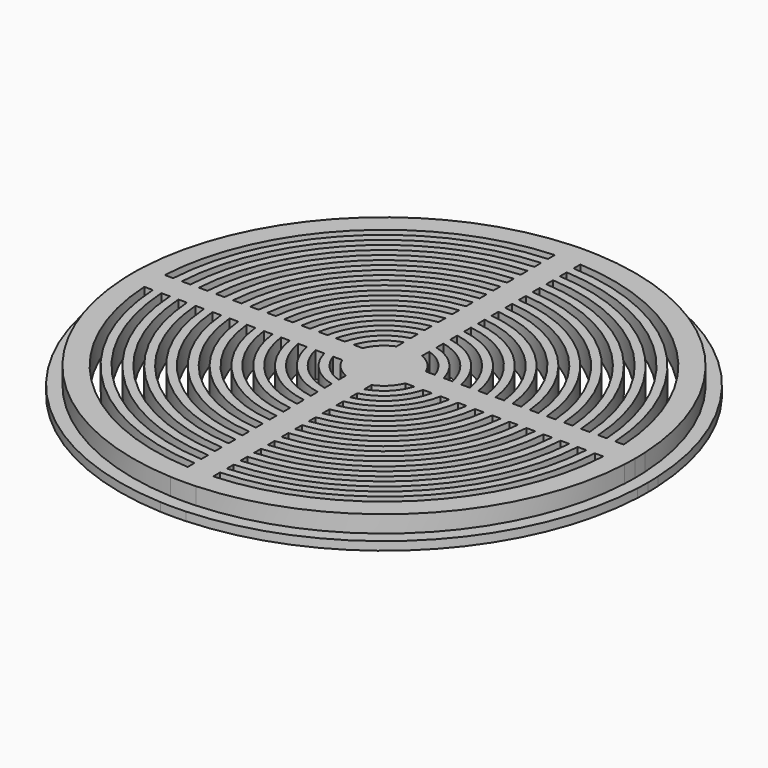
from build123d import *

# Parameters (mm, degrees)
F0_R     = 1
F1_DEPTH = 3
F2_DEPTH = 1


with BuildPart() as f1:
    # F0 (on Top) → F1 (new body)
    with BuildSketch(Plane.XY):
        with BuildLine():
            Line((-17.9373911147, 1.5), (-18.9406969249, 1.5))
            ThreePointArc((-18.9406969249, 1.5), (-19, 0), (-18.9406969249, -1.5))
            Line((-18.9406969249, -1.5), (-17.9373911147, -1.5))
            ThreePointArc((-17.9373911147, -1.5), (-18, 0), (-17.9373911147, 1.5))
        make_face()
        with BuildLine():
            Line((-11.9058808998, 1.5), (-12.9131715701, 1.5))
            ThreePointArc((-12.9131715701, 1.5), (-13, 0), (-12.9131715701, -1.5))
            Line((-12.9131715701, -1.5), (-11.9058808998, -1.5))
            ThreePointArc((-11.9058808998, -1.5), (-12, 0), (-11.9058808998, 1.5))
        make_face()
        with BuildLine():
            ThreePointArc((29.4618397253, -1.5), (29.4904583882, -0.7502426618), (29.5, 0))
            ThreePointArc((29.5, 0), (29.4904583882, 0.7502426618), (29.4618397253, 1.5))
            Line((29.4618397253, 1.5), (26.9583011334, 1.5))
            ThreePointArc((26.9583011334, 1.5), (26.9895732701, 0.7502897433), (27, 0))
            ThreePointArc((27, 0), (26.9895732701, -0.7502897433), (26.9583011334, -1.5))
            Line((26.9583011334, -1.5), (29.4618397253, -1.5))
        make_face()
        with BuildLine():
            ThreePointArc((26, 0), (25.9891714212, 0.750312493), (25.9566947048, 1.5))
            Line((25.9566947048, 1.5), (24.9549594269, 1.5))
            ThreePointArc((24.9549594269, 1.5), (24.9887373198, 0.7503380327), (25, 0))
            ThreePointArc((25, 0), (24.9887373198, -0.7503380327), (24.9549594269, -1.5))
            Line((24.9549594269, -1.5), (25.9566947048, -1.5))
            ThreePointArc((25.9566947048, -1.5), (25.9891714212, -0.750312493), (26, 0))
        make_face()
        with BuildLine():
            ThreePointArc((18, 0), (17.9843409674, 0.7506530278), (17.9373911147, 1.5))
            Line((17.9373911147, 1.5), (16.9336942219, 1.5))
            ThreePointArc((16.9336942219, 1.5), (16.9834154659, 0.7507323851), (17, 0))
            ThreePointArc((17, 0), (16.9834154659, -0.7507323851), (16.9336942219, -1.5))
            Line((16.9336942219, -1.5), (17.9373911147, -1.5))
            ThreePointArc((17.9373911147, -1.5), (17.9843409674, -0.7506530278), (18, 0))
        make_face()
        with BuildLine():
            Line((-19.9436706752, 1.5), (-20.9463600657, 1.5))
            ThreePointArc((-20.9463600657, 1.5), (-21, 0), (-20.9463600657, -1.5))
            Line((-20.9463600657, -1.5), (-19.9436706752, -1.5))
            ThreePointArc((-19.9436706752, -1.5), (-20, 0), (-19.9436706752, 1.5))
        make_face()
        with BuildLine():
            Line((-25.9566947048, 1.5), (-26.9583011334, 1.5))
            ThreePointArc((-26.9583011334, 1.5), (-27, 0), (-26.9583011334, -1.5))
            Line((-26.9583011334, -1.5), (-25.9566947048, -1.5))
            ThreePointArc((-25.9566947048, -1.5), (-26, 0), (-25.9566947048, 1.5))
        make_face()
        with BuildLine():
            Line((-1.5, 1.5), (-2.5980762114, 1.5))
            ThreePointArc((-2.5980762114, 1.5), (-3, 0), (-2.5980762114, -1.5))
            Line((-2.5980762114, -1.5), (-1.5, -1.5))
            Line((-1.5, -1.5), (-1.5, -1.3228756555))
            ThreePointArc((-1.5, -1.3228756555), (-2, 0), (-1.5, 1.3228756555))
            Line((-1.5, 1.3228756555), (-1.5, 1.5))
        make_face()
        with BuildLine():
            Line((-23.953079134, 1.5), (-24.9549594269, 1.5))
            ThreePointArc((-24.9549594269, 1.5), (-25, 0), (-24.9549594269, -1.5))
            Line((-24.9549594269, -1.5), (-23.953079134, -1.5))
            ThreePointArc((-23.953079134, -1.5), (-24, 0), (-23.953079134, 1.5))
        make_face()
        with BuildLine():
            Line((-21.9488040676, 1.5), (-22.9510348351, 1.5))
            ThreePointArc((-22.9510348351, 1.5), (-23, 0), (-22.9510348351, -1.5))
            Line((-22.9510348351, -1.5), (-21.9488040676, -1.5))
            ThreePointArc((-21.9488040676, -1.5), (-22, 0), (-21.9488040676, 1.5))
        make_face()
        with BuildLine():
            ThreePointArc((5, 0), (4.9420886291, 0.7587884964), (4.7696960071, 1.5))
            Line((4.7696960071, 1.5), (3.7080992435, 1.5))
            ThreePointArc((3.7080992435, 1.5), (3.92634671, 0.7640690498), (4, 0))
            ThreePointArc((4, 0), (3.92634671, -0.7640690498), (3.7080992435, -1.5))
            Line((3.7080992435, -1.5), (4.7696960071, -1.5))
            ThreePointArc((4.7696960071, -1.5), (4.9420886291, -0.7587884964), (5, 0))
        make_face()
        with BuildLine():
            Line((-7.8581168228, 1.5), (-8.8741196746, 1.5))
            ThreePointArc((-8.8741196746, 1.5), (-9, 0), (-8.8741196746, -1.5))
            Line((-8.8741196746, -1.5), (-7.8581168228, -1.5))
            ThreePointArc((-7.8581168228, -1.5), (-8, 0), (-7.8581168228, 1.5))
        make_face()
        with BuildLine():
            Line((-13.9194109071, 1.5), (-14.9248115566, 1.5))
            ThreePointArc((-14.9248115566, 1.5), (-15, 0), (-14.9248115566, -1.5))
            Line((-14.9248115566, -1.5), (-13.9194109071, -1.5))
            ThreePointArc((-13.9194109071, -1.5), (-14, 0), (-13.9194109071, 1.5))
        make_face()
        with BuildLine():
            Line((-15.9295323221, 1.5), (-16.9336942219, 1.5))
            ThreePointArc((-16.9336942219, 1.5), (-17, 0), (-16.9336942219, -1.5))
            Line((-16.9336942219, -1.5), (-15.9295323221, -1.5))
            ThreePointArc((-15.9295323221, -1.5), (-16, 0), (-15.9295323221, 1.5))
        make_face()
        with BuildLine():
            Line((-5.8094750193, 1.5), (-6.8373971656, 1.5))
            ThreePointArc((-6.8373971656, 1.5), (-7, 0), (-6.8373971656, -1.5))
            Line((-6.8373971656, -1.5), (-5.8094750193, -1.5))
            ThreePointArc((-5.8094750193, -1.5), (-6, 0), (-5.8094750193, 1.5))
        make_face()
        with BuildLine():
            ThreePointArc((3, 0), (2.8977774789, 0.7764571353), (2.5980762114, 1.5))
            Line((2.5980762114, 1.5), (1.5, 1.5))
            Line((1.5, 1.5), (1.5, 1.3228756555))
            ThreePointArc((1.5, 1.3228756555), (1.8708286934, 0.7071067812), (2, 0))
            ThreePointArc((2, 0), (1.8708286934, -0.7071067812), (1.5, -1.3228756555))
            Line((1.5, -1.3228756555), (1.5, -1.5))
            Line((1.5, -1.5), (2.5980762114, -1.5))
            ThreePointArc((2.5980762114, -1.5), (2.8977774789, -0.7764571353), (3, 0))
        make_face()
        with BuildLine():
            Line((-3.7080992435, 1.5), (-4.7696960071, 1.5))
            ThreePointArc((-4.7696960071, 1.5), (-5, 0), (-4.7696960071, -1.5))
            Line((-4.7696960071, -1.5), (-3.7080992435, -1.5))
            ThreePointArc((-3.7080992435, -1.5), (-4, 0), (-3.7080992435, 1.5))
        make_face()
        with BuildLine():
            Line((-9.8868599666, 1.5), (-10.8972473589, 1.5))
            ThreePointArc((-10.8972473589, 1.5), (-11, 0), (-10.8972473589, -1.5))
            Line((-10.8972473589, -1.5), (-9.8868599666, -1.5))
            ThreePointArc((-9.8868599666, -1.5), (-10, 0), (-9.8868599666, 1.5))
        make_face()
        with BuildLine():
            ThreePointArc((16, 0), (15.9823733712, 0.7508271595), (15.9295323221, 1.5))
            Line((15.9295323221, 1.5), (14.9248115566, 1.5))
            ThreePointArc((14.9248115566, 1.5), (14.9811910967, 0.7509416259), (15, 0))
            ThreePointArc((15, 0), (14.9811910967, -0.7509416259), (14.9248115566, -1.5))
            Line((14.9248115566, -1.5), (15.9295323221, -1.5))
            ThreePointArc((15.9295323221, -1.5), (15.9823733712, -0.7508271595), (16, 0))
        make_face()
        with BuildLine():
            ThreePointArc((4, 0), (3.92634671, 0.7640690498), (3.7080992435, 1.5))
            Line((3.7080992435, 1.5), (2.5980762114, 1.5))
            ThreePointArc((2.5980762114, 1.5), (2.8977774789, 0.7764571353), (3, 0))
            ThreePointArc((3, 0), (2.8977774789, -0.7764571353), (2.5980762114, -1.5))
            Line((2.5980762114, -1.5), (3.7080992435, -1.5))
            ThreePointArc((3.7080992435, -1.5), (3.92634671, -0.7640690498), (4, 0))
        make_face()
        with BuildLine():
            ThreePointArc((9, 0), (8.9684747051, 0.7526363425), (8.8741196746, 1.5))
            Line((8.8741196746, 1.5), (7.8581168228, 1.5))
            ThreePointArc((7.8581168228, 1.5), (7.964450219, 0.7533476681), (8, 0))
            ThreePointArc((8, 0), (7.964450219, -0.7533476681), (7.8581168228, -1.5))
            Line((7.8581168228, -1.5), (8.8741196746, -1.5))
            ThreePointArc((8.8741196746, -1.5), (8.9684747051, -0.7526363425), (9, 0))
        make_face()
        with BuildLine():
            ThreePointArc((12, 0), (11.9764471108, 0.7514749505), (11.9058808998, 1.5))
            Line((11.9058808998, 1.5), (10.8972473589, 1.5))
            ThreePointArc((10.8972473589, 1.5), (10.9742817748, 0.7517576247), (11, 0))
            ThreePointArc((11, 0), (10.9742817748, -0.7517576247), (10.8972473589, -1.5))
            Line((10.8972473589, -1.5), (11.9058808998, -1.5))
            ThreePointArc((11.9058808998, -1.5), (11.9764471108, -0.7514749505), (12, 0))
        make_face()
        with BuildLine():
            ThreePointArc((19, 0), (18.9851684424, 0.7505859136), (18.9406969249, 1.5))
            Line((18.9406969249, 1.5), (17.9373911147, 1.5))
            ThreePointArc((17.9373911147, 1.5), (17.9843409674, 0.7506530278), (18, 0))
            ThreePointArc((18, 0), (17.9843409674, -0.7506530278), (17.9373911147, -1.5))
            Line((17.9373911147, -1.5), (18.9406969249, -1.5))
            ThreePointArc((18.9406969249, -1.5), (18.9851684424, -0.7505859136), (19, 0))
        make_face()
        with BuildLine():
            ThreePointArc((7, 0), (6.9592305666, 0.7543937436), (6.8373971656, 1.5))
            Line((6.8373971656, 1.5), (5.8094750193, 1.5))
            ThreePointArc((5.8094750193, 1.5), (5.9521781776, 0.7560257549), (6, 0))
            ThreePointArc((6, 0), (5.9521781776, -0.7560257549), (5.8094750193, -1.5))
            Line((5.8094750193, -1.5), (6.8373971656, -1.5))
            ThreePointArc((6.8373971656, -1.5), (6.9592305666, -0.7543937436), (7, 0))
        make_face()
        with BuildLine():
            ThreePointArc((17, 0), (16.9834154659, 0.7507323851), (16.9336942219, 1.5))
            Line((16.9336942219, 1.5), (15.9295323221, 1.5))
            ThreePointArc((15.9295323221, 1.5), (15.9823733712, 0.7508271595), (16, 0))
            ThreePointArc((16, 0), (15.9823733712, -0.7508271595), (15.9295323221, -1.5))
            Line((15.9295323221, -1.5), (16.9336942219, -1.5))
            ThreePointArc((16.9336942219, -1.5), (16.9834154659, -0.7507323851), (17, 0))
        make_face()
        with BuildLine():
            ThreePointArc((6, 0), (5.9521781776, 0.7560257549), (5.8094750193, 1.5))
            Line((5.8094750193, 1.5), (4.7696960071, 1.5))
            ThreePointArc((4.7696960071, 1.5), (4.9420886291, 0.7587884964), (5, 0))
            ThreePointArc((5, 0), (4.9420886291, -0.7587884964), (4.7696960071, -1.5))
            Line((4.7696960071, -1.5), (5.8094750193, -1.5))
            ThreePointArc((5.8094750193, -1.5), (5.9521781776, -0.7560257549), (6, 0))
        make_face()
        with BuildLine():
            ThreePointArc((10, 0), (9.971674876, 0.7521304187), (9.8868599666, 1.5))
            Line((9.8868599666, 1.5), (8.8741196746, 1.5))
            ThreePointArc((8.8741196746, 1.5), (8.9684747051, 0.7526363425), (9, 0))
            ThreePointArc((9, 0), (8.9684747051, -0.7526363425), (8.8741196746, -1.5))
            Line((8.8741196746, -1.5), (9.8868599666, -1.5))
            ThreePointArc((9.8868599666, -1.5), (9.971674876, -0.7521304187), (10, 0))
        make_face()
        with BuildLine():
            ThreePointArc((8, 0), (7.964450219, 0.7533476681), (7.8581168228, 1.5))
            Line((7.8581168228, 1.5), (6.8373971656, 1.5))
            ThreePointArc((6.8373971656, 1.5), (6.9592305666, 0.7543937436), (7, 0))
            ThreePointArc((7, 0), (6.9592305666, -0.7543937436), (6.8373971656, -1.5))
            Line((6.8373971656, -1.5), (7.8581168228, -1.5))
            ThreePointArc((7.8581168228, -1.5), (7.964450219, -0.7533476681), (8, 0))
        make_face()
        with BuildLine():
            ThreePointArc((22, 0), (21.9871972917, 0.7504367101), (21.9488040676, 1.5))
            Line((21.9488040676, 1.5), (20.9463600657, 1.5))
            ThreePointArc((20.9463600657, 1.5), (20.9865857321, 0.7504793872), (21, 0))
            ThreePointArc((21, 0), (20.9865857321, -0.7504793872), (20.9463600657, -1.5))
            Line((20.9463600657, -1.5), (21.9488040676, -1.5))
            ThreePointArc((21.9488040676, -1.5), (21.9871972917, -0.7504367101), (22, 0))
        make_face()
        with BuildLine():
            ThreePointArc((20, 0), (19.9859127075, 0.7505286458), (19.9436706752, 1.5))
            Line((19.9436706752, 1.5), (18.9406969249, 1.5))
            ThreePointArc((18.9406969249, 1.5), (18.9851684424, 0.7505859136), (19, 0))
            ThreePointArc((19, 0), (18.9851684424, -0.7505859136), (18.9406969249, -1.5))
            Line((18.9406969249, -1.5), (19.9436706752, -1.5))
            ThreePointArc((19.9436706752, -1.5), (19.9859127075, -0.7505286458), (20, 0))
        make_face()
        with BuildLine():
            ThreePointArc((11, 0), (10.9742817748, 0.7517576247), (10.8972473589, 1.5))
            Line((10.8972473589, 1.5), (9.8868599666, 1.5))
            ThreePointArc((9.8868599666, 1.5), (9.971674876, 0.7521304187), (10, 0))
            ThreePointArc((10, 0), (9.971674876, -0.7521304187), (9.8868599666, -1.5))
            Line((9.8868599666, -1.5), (10.8972473589, -1.5))
            ThreePointArc((10.8972473589, -1.5), (10.9742817748, -0.7517576247), (11, 0))
        make_face()
        with BuildLine():
            ThreePointArc((14, 0), (13.979838209, 0.7510816537), (13.9194109071, 1.5))
            Line((13.9194109071, 1.5), (12.9131715701, 1.5))
            ThreePointArc((12.9131715701, 1.5), (12.9782747392, 0.7512554786), (13, 0))
            ThreePointArc((13, 0), (12.9782747392, -0.7512554786), (12.9131715701, -1.5))
            Line((12.9131715701, -1.5), (13.9194109071, -1.5))
            ThreePointArc((13.9194109071, -1.5), (13.979838209, -0.7510816537), (14, 0))
        make_face()
        with BuildLine():
            ThreePointArc((24, 0), (23.9882669155, 0.7503668382), (23.953079134, 1.5))
            Line((23.953079134, 1.5), (22.9510348351, 1.5))
            ThreePointArc((22.9510348351, 1.5), (22.9877554494, 0.7503994915), (23, 0))
            ThreePointArc((23, 0), (22.9877554494, -0.7503994915), (22.9510348351, -1.5))
            Line((22.9510348351, -1.5), (23.953079134, -1.5))
            ThreePointArc((23.953079134, -1.5), (23.9882669155, -0.7503668382), (24, 0))
        make_face()
        with BuildLine():
            ThreePointArc((21, 0), (20.9865857321, 0.7504793872), (20.9463600657, 1.5))
            Line((20.9463600657, 1.5), (19.9436706752, 1.5))
            ThreePointArc((19.9436706752, 1.5), (19.9859127075, 0.7505286458), (20, 0))
            ThreePointArc((20, 0), (19.9859127075, -0.7505286458), (19.9436706752, -1.5))
            Line((19.9436706752, -1.5), (20.9463600657, -1.5))
            ThreePointArc((20.9463600657, -1.5), (20.9865857321, -0.7504793872), (21, 0))
        make_face()
        with BuildLine():
            ThreePointArc((25, 0), (24.9887373198, 0.7503380327), (24.9549594269, 1.5))
            Line((24.9549594269, 1.5), (23.953079134, 1.5))
            ThreePointArc((23.953079134, 1.5), (23.9882669155, 0.7503668382), (24, 0))
            ThreePointArc((24, 0), (23.9882669155, -0.7503668382), (23.953079134, -1.5))
            Line((23.953079134, -1.5), (24.9549594269, -1.5))
            ThreePointArc((24.9549594269, -1.5), (24.9887373198, -0.7503380327), (25, 0))
        make_face()
        with BuildLine():
            ThreePointArc((23, 0), (22.9877554494, 0.7503994915), (22.9510348351, 1.5))
            Line((22.9510348351, 1.5), (21.9488040676, 1.5))
            ThreePointArc((21.9488040676, 1.5), (21.9871972917, 0.7504367101), (22, 0))
            ThreePointArc((22, 0), (21.9871972917, -0.7504367101), (21.9488040676, -1.5))
            Line((21.9488040676, -1.5), (22.9510348351, -1.5))
            ThreePointArc((22.9510348351, -1.5), (22.9877554494, -0.7503994915), (23, 0))
        make_face()
        with BuildLine():
            ThreePointArc((27, 0), (26.9895732701, 0.7502897433), (26.9583011334, 1.5))
            Line((26.9583011334, 1.5), (25.9566947048, 1.5))
            ThreePointArc((25.9566947048, 1.5), (25.9891714212, 0.750312493), (26, 0))
            ThreePointArc((26, 0), (25.9891714212, -0.750312493), (25.9566947048, -1.5))
            Line((25.9566947048, -1.5), (26.9583011334, -1.5))
            ThreePointArc((26.9583011334, -1.5), (26.9895732701, -0.7502897433), (27, 0))
        make_face()
        with BuildLine():
            ThreePointArc((15, 0), (14.9811910967, 0.7509416259), (14.9248115566, 1.5))
            Line((14.9248115566, 1.5), (13.9194109071, 1.5))
            ThreePointArc((13.9194109071, 1.5), (13.979838209, 0.7510816537), (14, 0))
            ThreePointArc((14, 0), (13.979838209, -0.7510816537), (13.9194109071, -1.5))
            Line((13.9194109071, -1.5), (14.9248115566, -1.5))
            ThreePointArc((14.9248115566, -1.5), (14.9811910967, -0.7509416259), (15, 0))
        make_face()
        with BuildLine():
            ThreePointArc((13, 0), (12.9782747392, 0.7512554786), (12.9131715701, 1.5))
            Line((12.9131715701, 1.5), (11.9058808998, 1.5))
            ThreePointArc((11.9058808998, 1.5), (11.9764471108, 0.7514749505), (12, 0))
            ThreePointArc((12, 0), (11.9764471108, -0.7514749505), (11.9058808998, -1.5))
            Line((11.9058808998, -1.5), (12.9131715701, -1.5))
            ThreePointArc((12.9131715701, -1.5), (12.9782747392, -0.7512554786), (13, 0))
        make_face()
        with BuildLine():
            Line((-18.9406969249, 1.5), (-19.9436706752, 1.5))
            ThreePointArc((-19.9436706752, 1.5), (-20, 0), (-19.9436706752, -1.5))
            Line((-19.9436706752, -1.5), (-18.9406969249, -1.5))
            ThreePointArc((-18.9406969249, -1.5), (-19, 0), (-18.9406969249, 1.5))
        make_face()
        with BuildLine():
            Line((-20.9463600657, 1.5), (-21.9488040676, 1.5))
            ThreePointArc((-21.9488040676, 1.5), (-22, 0), (-21.9488040676, -1.5))
            Line((-21.9488040676, -1.5), (-20.9463600657, -1.5))
            ThreePointArc((-20.9463600657, -1.5), (-21, 0), (-20.9463600657, 1.5))
        make_face()
        with BuildLine():
            Line((-22.9510348351, 1.5), (-23.953079134, 1.5))
            ThreePointArc((-23.953079134, 1.5), (-24, 0), (-23.953079134, -1.5))
            Line((-23.953079134, -1.5), (-22.9510348351, -1.5))
            ThreePointArc((-22.9510348351, -1.5), (-23, 0), (-22.9510348351, 1.5))
        make_face()
        with BuildLine():
            Line((-24.9549594269, 1.5), (-25.9566947048, 1.5))
            ThreePointArc((-25.9566947048, 1.5), (-26, 0), (-25.9566947048, -1.5))
            Line((-25.9566947048, -1.5), (-24.9549594269, -1.5))
            ThreePointArc((-24.9549594269, -1.5), (-25, 0), (-24.9549594269, 1.5))
        make_face()
        with BuildLine():
            Line((-10.8972473589, 1.5), (-11.9058808998, 1.5))
            ThreePointArc((-11.9058808998, 1.5), (-12, 0), (-11.9058808998, -1.5))
            Line((-11.9058808998, -1.5), (-10.8972473589, -1.5))
            ThreePointArc((-10.8972473589, -1.5), (-11, 0), (-10.8972473589, 1.5))
        make_face()
        with BuildLine():
            Line((-12.9131715701, 1.5), (-13.9194109071, 1.5))
            ThreePointArc((-13.9194109071, 1.5), (-14, 0), (-13.9194109071, -1.5))
            Line((-13.9194109071, -1.5), (-12.9131715701, -1.5))
            ThreePointArc((-12.9131715701, -1.5), (-13, 0), (-12.9131715701, 1.5))
        make_face()
        with BuildLine():
            Line((-14.9248115566, 1.5), (-15.9295323221, 1.5))
            ThreePointArc((-15.9295323221, 1.5), (-16, 0), (-15.9295323221, -1.5))
            Line((-15.9295323221, -1.5), (-14.9248115566, -1.5))
            ThreePointArc((-14.9248115566, -1.5), (-15, 0), (-14.9248115566, 1.5))
        make_face()
        with BuildLine():
            Line((-16.9336942219, 1.5), (-17.9373911147, 1.5))
            ThreePointArc((-17.9373911147, 1.5), (-18, 0), (-17.9373911147, -1.5))
            Line((-17.9373911147, -1.5), (-16.9336942219, -1.5))
            ThreePointArc((-16.9336942219, -1.5), (-17, 0), (-16.9336942219, 1.5))
        make_face()
        with BuildLine():
            Line((-2.5980762114, 1.5), (-3.7080992435, 1.5))
            ThreePointArc((-3.7080992435, 1.5), (-4, 0), (-3.7080992435, -1.5))
            Line((-3.7080992435, -1.5), (-2.5980762114, -1.5))
            ThreePointArc((-2.5980762114, -1.5), (-3, 0), (-2.5980762114, 1.5))
        make_face()
        with BuildLine():
            Line((-4.7696960071, 1.5), (-5.8094750193, 1.5))
            ThreePointArc((-5.8094750193, 1.5), (-6, 0), (-5.8094750193, -1.5))
            Line((-5.8094750193, -1.5), (-4.7696960071, -1.5))
            ThreePointArc((-4.7696960071, -1.5), (-5, 0), (-4.7696960071, 1.5))
        make_face()
        with BuildLine():
            Line((-6.8373971656, 1.5), (-7.8581168228, 1.5))
            ThreePointArc((-7.8581168228, 1.5), (-8, 0), (-7.8581168228, -1.5))
            Line((-7.8581168228, -1.5), (-6.8373971656, -1.5))
            ThreePointArc((-6.8373971656, -1.5), (-7, 0), (-6.8373971656, 1.5))
        make_face()
        with BuildLine():
            Line((-8.8741196746, 1.5), (-9.8868599666, 1.5))
            ThreePointArc((-9.8868599666, 1.5), (-10, 0), (-9.8868599666, -1.5))
            Line((-9.8868599666, -1.5), (-8.8741196746, -1.5))
            ThreePointArc((-8.8741196746, -1.5), (-9, 0), (-8.8741196746, 1.5))
        make_face()
        with BuildLine():
            Line((-26.9583011334, 1.5), (-29.4618397253, 1.5))
            ThreePointArc((-29.4618397253, 1.5), (-29.5, 0), (-29.4618397253, -1.5))
            Line((-29.4618397253, -1.5), (-26.9583011334, -1.5))
            ThreePointArc((-26.9583011334, -1.5), (-27, 0), (-26.9583011334, 1.5))
        make_face()
        with BuildLine():
            Line((1.5, -1.3228756555), (1.5, 1.3228756555))
            ThreePointArc((1.5, 1.3228756555), (1.4142135624, 1.4142135624), (1.3228756555, 1.5))
            Line((1.3228756555, 1.5), (-1.3228756555, 1.5))
            ThreePointArc((-1.3228756555, 1.5), (-1.4142135624, 1.4142135624), (-1.5, 1.3228756555))
            Line((-1.5, 1.3228756555), (-1.5, -1.3228756555))
            ThreePointArc((-1.5, -1.3228756555), (-1.4142135624, -1.4142135624), (-1.3228756555, -1.5))
            Line((-1.3228756555, -1.5), (1.3228756555, -1.5))
            ThreePointArc((1.3228756555, -1.5), (1.4142135624, -1.4142135624), (1.5, -1.3228756555))
        make_face()
        Circle(F0_R, mode=Mode.SUBTRACT)
        with BuildLine():
            Line((1.5, 1.3228756555), (1.5, 1.5))
            Line((1.5, 1.5), (1.3228756555, 1.5))
            ThreePointArc((1.3228756555, 1.5), (1.4142135624, 1.4142135624), (1.5, 1.3228756555))
        make_face()
        with BuildLine():
            ThreePointArc((2, 0), (1.8708286934, 0.7071067812), (1.5, 1.3228756555))
            Line((1.5, 1.3228756555), (1.5, -1.3228756555))
            ThreePointArc((1.5, -1.3228756555), (1.8708286934, -0.7071067812), (2, 0))
        make_face()
        with BuildLine():
            ThreePointArc((-1.3228756555, -1.5), (0, -2), (1.3228756555, -1.5))
            Line((1.3228756555, -1.5), (-1.3228756555, -1.5))
        make_face()
        with BuildLine():
            Line((-1.5, -1.3228756555), (-1.5, 1.3228756555))
            ThreePointArc((-1.5, 1.3228756555), (-2, 0), (-1.5, -1.3228756555))
        make_face()
        with BuildLine():
            Line((-1.3228756555, 1.5), (1.3228756555, 1.5))
            ThreePointArc((1.3228756555, 1.5), (0, 2), (-1.3228756555, 1.5))
        make_face()
        with BuildLine():
            Line((-1.5, -1.3228756555), (-1.5, -1.5))
            Line((-1.5, -1.5), (-1.3228756555, -1.5))
            ThreePointArc((-1.3228756555, -1.5), (-1.4142135624, -1.4142135624), (-1.5, -1.3228756555))
        make_face()
        with BuildLine():
            Line((-1.3228756555, 1.5), (-1.5, 1.5))
            Line((-1.5, 1.5), (-1.5, 1.3228756555))
            ThreePointArc((-1.5, 1.3228756555), (-1.4142135624, 1.4142135624), (-1.3228756555, 1.5))
        make_face()
        with BuildLine():
            Line((1.3228756555, -1.5), (1.5, -1.5))
            Line((1.5, -1.5), (1.5, -1.3228756555))
            ThreePointArc((1.5, -1.3228756555), (1.4142135624, -1.4142135624), (1.3228756555, -1.5))
        make_face()
        Circle(F0_R)
        with BuildLine():
            Line((1.5, 7.8581168228), (1.5, 8.8741196746))
            ThreePointArc((1.5, 8.8741196746), (0, 9), (-1.5, 8.8741196746))
            Line((-1.5, 8.8741196746), (-1.5, 7.8581168228))
            ThreePointArc((-1.5, 7.8581168228), (0, 8), (1.5, 7.8581168228))
        make_face()
        with BuildLine():
            ThreePointArc((-1.5, -6.8373971656), (0, -7), (1.5, -6.8373971656))
            Line((1.5, -6.8373971656), (1.5, -5.8094750193))
            ThreePointArc((1.5, -5.8094750193), (0, -6), (-1.5, -5.8094750193))
            Line((-1.5, -5.8094750193), (-1.5, -6.8373971656))
        make_face()
        with BuildLine():
            Line((1.5, 13.9194109071), (1.5, 14.9248115566))
            ThreePointArc((1.5, 14.9248115566), (0, 15), (-1.5, 14.9248115566))
            Line((-1.5, 14.9248115566), (-1.5, 13.9194109071))
            ThreePointArc((-1.5, 13.9194109071), (0, 14), (1.5, 13.9194109071))
        make_face()
        with BuildLine():
            Line((1.5, 3.7080992435), (1.5, 4.7696960071))
            ThreePointArc((1.5, 4.7696960071), (0, 5), (-1.5, 4.7696960071))
            Line((-1.5, 4.7696960071), (-1.5, 3.7080992435))
            ThreePointArc((-1.5, 3.7080992435), (0, 4), (1.5, 3.7080992435))
        make_face()
        with BuildLine():
            ThreePointArc((-1.5, -22.9510348351), (0, -23), (1.5, -22.9510348351))
            Line((1.5, -22.9510348351), (1.5, -21.9488040676))
            ThreePointArc((1.5, -21.9488040676), (0, -22), (-1.5, -21.9488040676))
            Line((-1.5, -21.9488040676), (-1.5, -22.9510348351))
        make_face()
        with BuildLine():
            Line((1.5, 9.8868599666), (1.5, 10.8972473589))
            ThreePointArc((1.5, 10.8972473589), (0, 11), (-1.5, 10.8972473589))
            Line((-1.5, 10.8972473589), (-1.5, 9.8868599666))
            ThreePointArc((-1.5, 9.8868599666), (0, 10), (1.5, 9.8868599666))
        make_face()
        with BuildLine():
            ThreePointArc((-1.5, -24.9549594269), (0, -25), (1.5, -24.9549594269))
            Line((1.5, -24.9549594269), (1.5, -23.953079134))
            ThreePointArc((1.5, -23.953079134), (0, -24), (-1.5, -23.953079134))
            Line((-1.5, -23.953079134), (-1.5, -24.9549594269))
        make_face()
        with BuildLine():
            ThreePointArc((-1.5, -10.8972473589), (0, -11), (1.5, -10.8972473589))
            Line((1.5, -10.8972473589), (1.5, -9.8868599666))
            ThreePointArc((1.5, -9.8868599666), (0, -10), (-1.5, -9.8868599666))
            Line((-1.5, -9.8868599666), (-1.5, -10.8972473589))
        make_face()
        with BuildLine():
            ThreePointArc((-1.5, -12.9131715701), (0, -13), (1.5, -12.9131715701))
            Line((1.5, -12.9131715701), (1.5, -11.9058808998))
            ThreePointArc((1.5, -11.9058808998), (0, -12), (-1.5, -11.9058808998))
            Line((-1.5, -11.9058808998), (-1.5, -12.9131715701))
        make_face()
        with BuildLine():
            ThreePointArc((-1.5, -2.5980762114), (0, -3), (1.5, -2.5980762114))
            Line((1.5, -2.5980762114), (1.5, -1.5))
            Line((1.5, -1.5), (1.3228756555, -1.5))
            ThreePointArc((1.3228756555, -1.5), (0, -2), (-1.3228756555, -1.5))
            Line((-1.3228756555, -1.5), (-1.5, -1.5))
            Line((-1.5, -1.5), (-1.5, -2.5980762114))
        make_face()
        with BuildLine():
            ThreePointArc((-1.5, -14.9248115566), (0, -15), (1.5, -14.9248115566))
            Line((1.5, -14.9248115566), (1.5, -13.9194109071))
            ThreePointArc((1.5, -13.9194109071), (0, -14), (-1.5, -13.9194109071))
            Line((-1.5, -13.9194109071), (-1.5, -14.9248115566))
        make_face()
        with BuildLine():
            ThreePointArc((-1.5, -4.7696960071), (0, -5), (1.5, -4.7696960071))
            Line((1.5, -4.7696960071), (1.5, -3.7080992435))
            ThreePointArc((1.5, -3.7080992435), (0, -4), (-1.5, -3.7080992435))
            Line((-1.5, -3.7080992435), (-1.5, -4.7696960071))
        make_face()
        with BuildLine():
            ThreePointArc((-1.5, -8.8741196746), (0, -9), (1.5, -8.8741196746))
            Line((1.5, -8.8741196746), (1.5, -7.8581168228))
            ThreePointArc((1.5, -7.8581168228), (0, -8), (-1.5, -7.8581168228))
            Line((-1.5, -7.8581168228), (-1.5, -8.8741196746))
        make_face()
        with BuildLine():
            Line((1.5, 11.9058808998), (1.5, 12.9131715701))
            ThreePointArc((1.5, 12.9131715701), (0, 13), (-1.5, 12.9131715701))
            Line((-1.5, 12.9131715701), (-1.5, 11.9058808998))
            ThreePointArc((-1.5, 11.9058808998), (0, 12), (1.5, 11.9058808998))
        make_face()
        with BuildLine():
            Line((1.5, 25.9566947048), (1.5, 26.9583011334))
            ThreePointArc((1.5, 26.9583011334), (0, 27), (-1.5, 26.9583011334))
            Line((-1.5, 26.9583011334), (-1.5, 25.9566947048))
            ThreePointArc((-1.5, 25.9566947048), (0, 26), (1.5, 25.9566947048))
        make_face()
        with BuildLine():
            ThreePointArc((-1.5, -20.9463600657), (0, -21), (1.5, -20.9463600657))
            Line((1.5, -20.9463600657), (1.5, -19.9436706752))
            ThreePointArc((1.5, -19.9436706752), (0, -20), (-1.5, -19.9436706752))
            Line((-1.5, -19.9436706752), (-1.5, -20.9463600657))
        make_face()
        with BuildLine():
            ThreePointArc((-1.5, -16.9336942219), (0, -17), (1.5, -16.9336942219))
            Line((1.5, -16.9336942219), (1.5, -15.9295323221))
            ThreePointArc((1.5, -15.9295323221), (0, -16), (-1.5, -15.9295323221))
            Line((-1.5, -15.9295323221), (-1.5, -16.9336942219))
        make_face()
        with BuildLine():
            ThreePointArc((-1.5, -26.9583011334), (0, -27), (1.5, -26.9583011334))
            Line((1.5, -26.9583011334), (1.5, -25.9566947048))
            ThreePointArc((1.5, -25.9566947048), (0, -26), (-1.5, -25.9566947048))
            Line((-1.5, -25.9566947048), (-1.5, -26.9583011334))
        make_face()
        with BuildLine():
            Line((1.5, 5.8094750193), (1.5, 6.8373971656))
            ThreePointArc((1.5, 6.8373971656), (0, 7), (-1.5, 6.8373971656))
            Line((-1.5, 6.8373971656), (-1.5, 5.8094750193))
            ThreePointArc((-1.5, 5.8094750193), (0, 6), (1.5, 5.8094750193))
        make_face()
        with BuildLine():
            Line((1.5, 19.9436706752), (1.5, 20.9463600657))
            ThreePointArc((1.5, 20.9463600657), (0, 21), (-1.5, 20.9463600657))
            Line((-1.5, 20.9463600657), (-1.5, 19.9436706752))
            ThreePointArc((-1.5, 19.9436706752), (0, 20), (1.5, 19.9436706752))
        make_face()
        with BuildLine():
            ThreePointArc((-1.5, -18.9406969249), (0, -19), (1.5, -18.9406969249))
            Line((1.5, -18.9406969249), (1.5, -17.9373911147))
            ThreePointArc((1.5, -17.9373911147), (0, -18), (-1.5, -17.9373911147))
            Line((-1.5, -17.9373911147), (-1.5, -18.9406969249))
        make_face()
        with BuildLine():
            Line((1.5, 17.9373911147), (1.5, 18.9406969249))
            ThreePointArc((1.5, 18.9406969249), (0, 19), (-1.5, 18.9406969249))
            Line((-1.5, 18.9406969249), (-1.5, 17.9373911147))
            ThreePointArc((-1.5, 17.9373911147), (0, 18), (1.5, 17.9373911147))
        make_face()
        with BuildLine():
            Line((1.5, 15.9295323221), (1.5, 16.9336942219))
            ThreePointArc((1.5, 16.9336942219), (0, 17), (-1.5, 16.9336942219))
            Line((-1.5, 16.9336942219), (-1.5, 15.9295323221))
            ThreePointArc((-1.5, 15.9295323221), (0, 16), (1.5, 15.9295323221))
        make_face()
        with BuildLine():
            Line((1.5, 21.9488040676), (1.5, 22.9510348351))
            ThreePointArc((1.5, 22.9510348351), (0, 23), (-1.5, 22.9510348351))
            Line((-1.5, 22.9510348351), (-1.5, 21.9488040676))
            ThreePointArc((-1.5, 21.9488040676), (0, 22), (1.5, 21.9488040676))
        make_face()
        with BuildLine():
            Line((1.5, 20.9463600657), (1.5, 21.9488040676))
            ThreePointArc((1.5, 21.9488040676), (0, 22), (-1.5, 21.9488040676))
            Line((-1.5, 21.9488040676), (-1.5, 20.9463600657))
            ThreePointArc((-1.5, 20.9463600657), (0, 21), (1.5, 20.9463600657))
        make_face()
        with BuildLine():
            Line((1.5, 22.9510348351), (1.5, 23.953079134))
            ThreePointArc((1.5, 23.953079134), (0, 24), (-1.5, 23.953079134))
            Line((-1.5, 23.953079134), (-1.5, 22.9510348351))
            ThreePointArc((-1.5, 22.9510348351), (0, 23), (1.5, 22.9510348351))
        make_face()
        with BuildLine():
            Line((1.5, 23.953079134), (1.5, 24.9549594269))
            ThreePointArc((1.5, 24.9549594269), (0, 25), (-1.5, 24.9549594269))
            Line((-1.5, 24.9549594269), (-1.5, 23.953079134))
            ThreePointArc((-1.5, 23.953079134), (0, 24), (1.5, 23.953079134))
        make_face()
        with BuildLine():
            Line((1.5, 18.9406969249), (1.5, 19.9436706752))
            ThreePointArc((1.5, 19.9436706752), (0, 20), (-1.5, 19.9436706752))
            Line((-1.5, 19.9436706752), (-1.5, 18.9406969249))
            ThreePointArc((-1.5, 18.9406969249), (0, 19), (1.5, 18.9406969249))
        make_face()
        with BuildLine():
            ThreePointArc((-1.5, -29.4618397253), (0, -29.5), (1.5, -29.4618397253))
            Line((1.5, -29.4618397253), (1.5, -26.9583011334))
            ThreePointArc((1.5, -26.9583011334), (0, -27), (-1.5, -26.9583011334))
            Line((-1.5, -26.9583011334), (-1.5, -29.4618397253))
        make_face()
        with BuildLine():
            Line((1.5, 24.9549594269), (1.5, 25.9566947048))
            ThreePointArc((1.5, 25.9566947048), (0, 26), (-1.5, 25.9566947048))
            Line((-1.5, 25.9566947048), (-1.5, 24.9549594269))
            ThreePointArc((-1.5, 24.9549594269), (0, 25), (1.5, 24.9549594269))
        make_face()
        with BuildLine():
            Line((1.5, 10.8972473589), (1.5, 11.9058808998))
            ThreePointArc((1.5, 11.9058808998), (0, 12), (-1.5, 11.9058808998))
            Line((-1.5, 11.9058808998), (-1.5, 10.8972473589))
            ThreePointArc((-1.5, 10.8972473589), (0, 11), (1.5, 10.8972473589))
        make_face()
        with BuildLine():
            Line((1.5, 12.9131715701), (1.5, 13.9194109071))
            ThreePointArc((1.5, 13.9194109071), (0, 14), (-1.5, 13.9194109071))
            Line((-1.5, 13.9194109071), (-1.5, 12.9131715701))
            ThreePointArc((-1.5, 12.9131715701), (0, 13), (1.5, 12.9131715701))
        make_face()
        with BuildLine():
            Line((1.5, 14.9248115566), (1.5, 15.9295323221))
            ThreePointArc((1.5, 15.9295323221), (0, 16), (-1.5, 15.9295323221))
            Line((-1.5, 15.9295323221), (-1.5, 14.9248115566))
            ThreePointArc((-1.5, 14.9248115566), (0, 15), (1.5, 14.9248115566))
        make_face()
        with BuildLine():
            Line((1.5, 16.9336942219), (1.5, 17.9373911147))
            ThreePointArc((1.5, 17.9373911147), (0, 18), (-1.5, 17.9373911147))
            Line((-1.5, 17.9373911147), (-1.5, 16.9336942219))
            ThreePointArc((-1.5, 16.9336942219), (0, 17), (1.5, 16.9336942219))
        make_face()
        with BuildLine():
            Line((1.5, 2.5980762114), (1.5, 3.7080992435))
            ThreePointArc((1.5, 3.7080992435), (0, 4), (-1.5, 3.7080992435))
            Line((-1.5, 3.7080992435), (-1.5, 2.5980762114))
            ThreePointArc((-1.5, 2.5980762114), (0, 3), (1.5, 2.5980762114))
        make_face()
        with BuildLine():
            Line((1.5, 4.7696960071), (1.5, 5.8094750193))
            ThreePointArc((1.5, 5.8094750193), (0, 6), (-1.5, 5.8094750193))
            Line((-1.5, 5.8094750193), (-1.5, 4.7696960071))
            ThreePointArc((-1.5, 4.7696960071), (0, 5), (1.5, 4.7696960071))
        make_face()
        with BuildLine():
            Line((1.5, 6.8373971656), (1.5, 7.8581168228))
            ThreePointArc((1.5, 7.8581168228), (0, 8), (-1.5, 7.8581168228))
            Line((-1.5, 7.8581168228), (-1.5, 6.8373971656))
            ThreePointArc((-1.5, 6.8373971656), (0, 7), (1.5, 6.8373971656))
        make_face()
        with BuildLine():
            Line((1.5, 8.8741196746), (1.5, 9.8868599666))
            ThreePointArc((1.5, 9.8868599666), (0, 10), (-1.5, 9.8868599666))
            Line((-1.5, 9.8868599666), (-1.5, 8.8741196746))
            ThreePointArc((-1.5, 8.8741196746), (0, 9), (1.5, 8.8741196746))
        make_face()
        with BuildLine():
            Line((1.5, 26.9583011334), (1.5, 29.4618397253))
            ThreePointArc((1.5, 29.4618397253), (0, 29.5), (-1.5, 29.4618397253))
            Line((-1.5, 29.4618397253), (-1.5, 26.9583011334))
            ThreePointArc((-1.5, 26.9583011334), (0, 27), (1.5, 26.9583011334))
        make_face()
        with BuildLine():
            ThreePointArc((-1.5, -15.9295323221), (0, -16), (1.5, -15.9295323221))
            Line((1.5, -15.9295323221), (1.5, -14.9248115566))
            ThreePointArc((1.5, -14.9248115566), (0, -15), (-1.5, -14.9248115566))
            Line((-1.5, -14.9248115566), (-1.5, -15.9295323221))
        make_face()
        with BuildLine():
            ThreePointArc((-1.5, -17.9373911147), (0, -18), (1.5, -17.9373911147))
            Line((1.5, -17.9373911147), (1.5, -16.9336942219))
            ThreePointArc((1.5, -16.9336942219), (0, -17), (-1.5, -16.9336942219))
            Line((-1.5, -16.9336942219), (-1.5, -17.9373911147))
        make_face()
        with BuildLine():
            ThreePointArc((-1.5, -19.9436706752), (0, -20), (1.5, -19.9436706752))
            Line((1.5, -19.9436706752), (1.5, -18.9406969249))
            ThreePointArc((1.5, -18.9406969249), (0, -19), (-1.5, -18.9406969249))
            Line((-1.5, -18.9406969249), (-1.5, -19.9436706752))
        make_face()
        with BuildLine():
            ThreePointArc((-1.5, -21.9488040676), (0, -22), (1.5, -21.9488040676))
            Line((1.5, -21.9488040676), (1.5, -20.9463600657))
            ThreePointArc((1.5, -20.9463600657), (0, -21), (-1.5, -20.9463600657))
            Line((-1.5, -20.9463600657), (-1.5, -21.9488040676))
        make_face()
        with BuildLine():
            ThreePointArc((-1.5, -7.8581168228), (0, -8), (1.5, -7.8581168228))
            Line((1.5, -7.8581168228), (1.5, -6.8373971656))
            ThreePointArc((1.5, -6.8373971656), (0, -7), (-1.5, -6.8373971656))
            Line((-1.5, -6.8373971656), (-1.5, -7.8581168228))
        make_face()
        with BuildLine():
            ThreePointArc((-1.5, -9.8868599666), (0, -10), (1.5, -9.8868599666))
            Line((1.5, -9.8868599666), (1.5, -8.8741196746))
            ThreePointArc((1.5, -8.8741196746), (0, -9), (-1.5, -8.8741196746))
            Line((-1.5, -8.8741196746), (-1.5, -9.8868599666))
        make_face()
        with BuildLine():
            ThreePointArc((-1.5, -11.9058808998), (0, -12), (1.5, -11.9058808998))
            Line((1.5, -11.9058808998), (1.5, -10.8972473589))
            ThreePointArc((1.5, -10.8972473589), (0, -11), (-1.5, -10.8972473589))
            Line((-1.5, -10.8972473589), (-1.5, -11.9058808998))
        make_face()
        with BuildLine():
            ThreePointArc((-1.5, -13.9194109071), (0, -14), (1.5, -13.9194109071))
            Line((1.5, -13.9194109071), (1.5, -12.9131715701))
            ThreePointArc((1.5, -12.9131715701), (0, -13), (-1.5, -12.9131715701))
            Line((-1.5, -12.9131715701), (-1.5, -13.9194109071))
        make_face()
        with BuildLine():
            ThreePointArc((-1.5, -3.7080992435), (0, -4), (1.5, -3.7080992435))
            Line((1.5, -3.7080992435), (1.5, -2.5980762114))
            ThreePointArc((1.5, -2.5980762114), (0, -3), (-1.5, -2.5980762114))
            Line((-1.5, -2.5980762114), (-1.5, -3.7080992435))
        make_face()
        with BuildLine():
            ThreePointArc((-1.5, -5.8094750193), (0, -6), (1.5, -5.8094750193))
            Line((1.5, -5.8094750193), (1.5, -4.7696960071))
            ThreePointArc((1.5, -4.7696960071), (0, -5), (-1.5, -4.7696960071))
            Line((-1.5, -4.7696960071), (-1.5, -5.8094750193))
        make_face()
        with BuildLine():
            ThreePointArc((-1.5, -23.953079134), (0, -24), (1.5, -23.953079134))
            Line((1.5, -23.953079134), (1.5, -22.9510348351))
            ThreePointArc((1.5, -22.9510348351), (0, -23), (-1.5, -22.9510348351))
            Line((-1.5, -22.9510348351), (-1.5, -23.953079134))
        make_face()
        with BuildLine():
            ThreePointArc((-1.5, -25.9566947048), (0, -26), (1.5, -25.9566947048))
            Line((1.5, -25.9566947048), (1.5, -24.9549594269))
            ThreePointArc((1.5, -24.9549594269), (0, -25), (-1.5, -24.9549594269))
            Line((-1.5, -24.9549594269), (-1.5, -25.9566947048))
        make_face()
        with BuildLine():
            Line((1.5, 1.5), (1.5, 2.5980762114))
            ThreePointArc((1.5, 2.5980762114), (0, 3), (-1.5, 2.5980762114))
            Line((-1.5, 2.5980762114), (-1.5, 1.5))
            Line((-1.5, 1.5), (-1.3228756555, 1.5))
            ThreePointArc((-1.3228756555, 1.5), (0, 2), (1.3228756555, 1.5))
            Line((1.3228756555, 1.5), (1.5, 1.5))
        make_face()
        with BuildLine():
            Line((-1.5, 1.5), (-1.5, 2.5980762114))
            ThreePointArc((-1.5, 2.5980762114), (-2.1213203436, 2.1213203436), (-2.5980762114, 1.5))
            Line((-2.5980762114, 1.5), (-1.5, 1.5))
        make_face()
        with BuildLine():
            ThreePointArc((-3.7080992435, -1.5), (-2.8284271247, -2.8284271247), (-1.5, -3.7080992435))
            Line((-1.5, -3.7080992435), (-1.5, -2.5980762114))
            ThreePointArc((-1.5, -2.5980762114), (-2.1213203436, -2.1213203436), (-2.5980762114, -1.5))
            Line((-2.5980762114, -1.5), (-3.7080992435, -1.5))
        make_face()
        with BuildLine():
            ThreePointArc((-2.5980762114, -1.5), (-2.1213203436, -2.1213203436), (-1.5, -2.5980762114))
            Line((-1.5, -2.5980762114), (-1.5, -1.5))
            Line((-1.5, -1.5), (-2.5980762114, -1.5))
        make_face()
        with BuildLine():
            Line((-1.5, 2.5980762114), (-1.5, 3.7080992435))
            ThreePointArc((-1.5, 3.7080992435), (-2.8284271247, 2.8284271247), (-3.7080992435, 1.5))
            Line((-3.7080992435, 1.5), (-2.5980762114, 1.5))
            ThreePointArc((-2.5980762114, 1.5), (-2.1213203436, 2.1213203436), (-1.5, 2.5980762114))
        make_face()
        with BuildLine():
            Line((2.5980762114, 1.5), (3.7080992435, 1.5))
            ThreePointArc((3.7080992435, 1.5), (2.8284271247, 2.8284271247), (1.5, 3.7080992435))
            Line((1.5, 3.7080992435), (1.5, 2.5980762114))
            ThreePointArc((1.5, 2.5980762114), (2.1213203436, 2.1213203436), (2.5980762114, 1.5))
        make_face()
        with BuildLine():
            Line((1.5, 1.5), (2.5980762114, 1.5))
            ThreePointArc((2.5980762114, 1.5), (2.1213203436, 2.1213203436), (1.5, 2.5980762114))
            Line((1.5, 2.5980762114), (1.5, 1.5))
        make_face()
        with BuildLine():
            ThreePointArc((1.5, -2.5980762114), (2.1213203436, -2.1213203436), (2.5980762114, -1.5))
            Line((2.5980762114, -1.5), (1.5, -1.5))
            Line((1.5, -1.5), (1.5, -2.5980762114))
        make_face()
        with BuildLine():
            ThreePointArc((1.5, -3.7080992435), (2.8284271247, -2.8284271247), (3.7080992435, -1.5))
            Line((3.7080992435, -1.5), (2.5980762114, -1.5))
            ThreePointArc((2.5980762114, -1.5), (2.1213203436, -2.1213203436), (1.5, -2.5980762114))
            Line((1.5, -2.5980762114), (1.5, -3.7080992435))
        make_face()
        with BuildLine():
            Line((-1.5, 4.7696960071), (-1.5, 5.8094750193))
            ThreePointArc((-1.5, 5.8094750193), (-4.2426406871, 4.2426406871), (-5.8094750193, 1.5))
            Line((-5.8094750193, 1.5), (-4.7696960071, 1.5))
            ThreePointArc((-4.7696960071, 1.5), (-3.5355339059, 3.5355339059), (-1.5, 4.7696960071))
        make_face()
        with BuildLine():
            Line((-1.5, 6.8373971656), (-1.5, 7.8581168228))
            ThreePointArc((-1.5, 7.8581168228), (-5.6568542495, 5.6568542495), (-7.8581168228, 1.5))
            Line((-7.8581168228, 1.5), (-6.8373971656, 1.5))
            ThreePointArc((-6.8373971656, 1.5), (-4.9497474683, 4.9497474683), (-1.5, 6.8373971656))
        make_face()
        with BuildLine():
            Line((-1.5, 8.8741196746), (-1.5, 9.8868599666))
            ThreePointArc((-1.5, 9.8868599666), (-7.0710678119, 7.0710678119), (-9.8868599666, 1.5))
            Line((-9.8868599666, 1.5), (-8.8741196746, 1.5))
            ThreePointArc((-8.8741196746, 1.5), (-6.3639610307, 6.3639610307), (-1.5, 8.8741196746))
        make_face()
        with BuildLine():
            Line((-1.5, 10.8972473589), (-1.5, 11.9058808998))
            ThreePointArc((-1.5, 11.9058808998), (-8.4852813742, 8.4852813742), (-11.9058808998, 1.5))
            Line((-11.9058808998, 1.5), (-10.8972473589, 1.5))
            ThreePointArc((-10.8972473589, 1.5), (-7.7781745931, 7.7781745931), (-1.5, 10.8972473589))
        make_face()
        with BuildLine():
            Line((-1.5, 12.9131715701), (-1.5, 13.9194109071))
            ThreePointArc((-1.5, 13.9194109071), (-9.8994949366, 9.8994949366), (-13.9194109071, 1.5))
            Line((-13.9194109071, 1.5), (-12.9131715701, 1.5))
            ThreePointArc((-12.9131715701, 1.5), (-9.1923881554, 9.1923881554), (-1.5, 12.9131715701))
        make_face()
        with BuildLine():
            Line((-1.5, 14.9248115566), (-1.5, 15.9295323221))
            ThreePointArc((-1.5, 15.9295323221), (-11.313708499, 11.313708499), (-15.9295323221, 1.5))
            Line((-15.9295323221, 1.5), (-14.9248115566, 1.5))
            ThreePointArc((-14.9248115566, 1.5), (-10.6066017178, 10.6066017178), (-1.5, 14.9248115566))
        make_face()
        with BuildLine():
            Line((-1.5, 16.9336942219), (-1.5, 17.9373911147))
            ThreePointArc((-1.5, 17.9373911147), (-12.7279220614, 12.7279220614), (-17.9373911147, 1.5))
            Line((-17.9373911147, 1.5), (-16.9336942219, 1.5))
            ThreePointArc((-16.9336942219, 1.5), (-12.0208152802, 12.0208152802), (-1.5, 16.9336942219))
        make_face()
        with BuildLine():
            Line((-1.5, 18.9406969249), (-1.5, 19.9436706752))
            ThreePointArc((-1.5, 19.9436706752), (-14.1421356237, 14.1421356237), (-19.9436706752, 1.5))
            Line((-19.9436706752, 1.5), (-18.9406969249, 1.5))
            ThreePointArc((-18.9406969249, 1.5), (-13.4350288425, 13.4350288425), (-1.5, 18.9406969249))
        make_face()
        with BuildLine():
            Line((-1.5, 20.9463600657), (-1.5, 21.9488040676))
            ThreePointArc((-1.5, 21.9488040676), (-15.5563491861, 15.5563491861), (-21.9488040676, 1.5))
            Line((-21.9488040676, 1.5), (-20.9463600657, 1.5))
            ThreePointArc((-20.9463600657, 1.5), (-14.8492424049, 14.8492424049), (-1.5, 20.9463600657))
        make_face()
        with BuildLine():
            Line((-1.5, 22.9510348351), (-1.5, 23.953079134))
            ThreePointArc((-1.5, 23.953079134), (-16.9705627485, 16.9705627485), (-23.953079134, 1.5))
            Line((-23.953079134, 1.5), (-22.9510348351, 1.5))
            ThreePointArc((-22.9510348351, 1.5), (-16.2634559673, 16.2634559673), (-1.5, 22.9510348351))
        make_face()
        with BuildLine():
            Line((-1.5, 24.9549594269), (-1.5, 25.9566947048))
            ThreePointArc((-1.5, 25.9566947048), (-18.3847763109, 18.3847763109), (-25.9566947048, 1.5))
            Line((-25.9566947048, 1.5), (-24.9549594269, 1.5))
            ThreePointArc((-24.9549594269, 1.5), (-17.6776695297, 17.6776695297), (-1.5, 24.9549594269))
        make_face()
        with BuildLine():
            Line((4.7696960071, 1.5), (5.8094750193, 1.5))
            ThreePointArc((5.8094750193, 1.5), (4.2426406871, 4.2426406871), (1.5, 5.8094750193))
            Line((1.5, 5.8094750193), (1.5, 4.7696960071))
            ThreePointArc((1.5, 4.7696960071), (3.5355339059, 3.5355339059), (4.7696960071, 1.5))
        make_face()
        with BuildLine():
            Line((6.8373971656, 1.5), (7.8581168228, 1.5))
            ThreePointArc((7.8581168228, 1.5), (5.6568542495, 5.6568542495), (1.5, 7.8581168228))
            Line((1.5, 7.8581168228), (1.5, 6.8373971656))
            ThreePointArc((1.5, 6.8373971656), (4.9497474683, 4.9497474683), (6.8373971656, 1.5))
        make_face()
        with BuildLine():
            Line((8.8741196746, 1.5), (9.8868599666, 1.5))
            ThreePointArc((9.8868599666, 1.5), (7.0710678119, 7.0710678119), (1.5, 9.8868599666))
            Line((1.5, 9.8868599666), (1.5, 8.8741196746))
            ThreePointArc((1.5, 8.8741196746), (6.3639610307, 6.3639610307), (8.8741196746, 1.5))
        make_face()
        with BuildLine():
            Line((10.8972473589, 1.5), (11.9058808998, 1.5))
            ThreePointArc((11.9058808998, 1.5), (8.4852813742, 8.4852813742), (1.5, 11.9058808998))
            Line((1.5, 11.9058808998), (1.5, 10.8972473589))
            ThreePointArc((1.5, 10.8972473589), (7.7781745931, 7.7781745931), (10.8972473589, 1.5))
        make_face()
        with BuildLine():
            Line((12.9131715701, 1.5), (13.9194109071, 1.5))
            ThreePointArc((13.9194109071, 1.5), (9.8994949366, 9.8994949366), (1.5, 13.9194109071))
            Line((1.5, 13.9194109071), (1.5, 12.9131715701))
            ThreePointArc((1.5, 12.9131715701), (9.1923881554, 9.1923881554), (12.9131715701, 1.5))
        make_face()
        with BuildLine():
            Line((14.9248115566, 1.5), (15.9295323221, 1.5))
            ThreePointArc((15.9295323221, 1.5), (11.313708499, 11.313708499), (1.5, 15.9295323221))
            Line((1.5, 15.9295323221), (1.5, 14.9248115566))
            ThreePointArc((1.5, 14.9248115566), (10.6066017178, 10.6066017178), (14.9248115566, 1.5))
        make_face()
        with BuildLine():
            Line((16.9336942219, 1.5), (17.9373911147, 1.5))
            ThreePointArc((17.9373911147, 1.5), (12.7279220614, 12.7279220614), (1.5, 17.9373911147))
            Line((1.5, 17.9373911147), (1.5, 16.9336942219))
            ThreePointArc((1.5, 16.9336942219), (12.0208152802, 12.0208152802), (16.9336942219, 1.5))
        make_face()
        with BuildLine():
            Line((18.9406969249, 1.5), (19.9436706752, 1.5))
            ThreePointArc((19.9436706752, 1.5), (14.1421356237, 14.1421356237), (1.5, 19.9436706752))
            Line((1.5, 19.9436706752), (1.5, 18.9406969249))
            ThreePointArc((1.5, 18.9406969249), (13.4350288425, 13.4350288425), (18.9406969249, 1.5))
        make_face()
        with BuildLine():
            Line((20.9463600657, 1.5), (21.9488040676, 1.5))
            ThreePointArc((21.9488040676, 1.5), (15.5563491861, 15.5563491861), (1.5, 21.9488040676))
            Line((1.5, 21.9488040676), (1.5, 20.9463600657))
            ThreePointArc((1.5, 20.9463600657), (14.8492424049, 14.8492424049), (20.9463600657, 1.5))
        make_face()
        with BuildLine():
            Line((22.9510348351, 1.5), (23.953079134, 1.5))
            ThreePointArc((23.953079134, 1.5), (16.9705627485, 16.9705627485), (1.5, 23.953079134))
            Line((1.5, 23.953079134), (1.5, 22.9510348351))
            ThreePointArc((1.5, 22.9510348351), (16.2634559673, 16.2634559673), (22.9510348351, 1.5))
        make_face()
        with BuildLine():
            Line((24.9549594269, 1.5), (25.9566947048, 1.5))
            ThreePointArc((25.9566947048, 1.5), (18.3847763108, 18.3847763109), (1.5, 25.9566947048))
            Line((1.5, 25.9566947048), (1.5, 24.9549594269))
            ThreePointArc((1.5, 24.9549594269), (17.6776695297, 17.6776695297), (24.9549594269, 1.5))
        make_face()
        with BuildLine():
            ThreePointArc((1.5, -5.8094750193), (4.2426406871, -4.2426406871), (5.8094750193, -1.5))
            Line((5.8094750193, -1.5), (4.7696960071, -1.5))
            ThreePointArc((4.7696960071, -1.5), (3.5355339059, -3.5355339059), (1.5, -4.7696960071))
            Line((1.5, -4.7696960071), (1.5, -5.8094750193))
        make_face()
        with BuildLine():
            ThreePointArc((1.5, -7.8581168228), (5.6568542495, -5.6568542495), (7.8581168228, -1.5))
            Line((7.8581168228, -1.5), (6.8373971656, -1.5))
            ThreePointArc((6.8373971656, -1.5), (4.9497474683, -4.9497474683), (1.5, -6.8373971656))
            Line((1.5, -6.8373971656), (1.5, -7.8581168228))
        make_face()
        with BuildLine():
            ThreePointArc((1.5, -9.8868599666), (7.0710678119, -7.0710678119), (9.8868599666, -1.5))
            Line((9.8868599666, -1.5), (8.8741196746, -1.5))
            ThreePointArc((8.8741196746, -1.5), (6.3639610307, -6.3639610307), (1.5, -8.8741196746))
            Line((1.5, -8.8741196746), (1.5, -9.8868599666))
        make_face()
        with BuildLine():
            ThreePointArc((1.5, -11.9058808998), (8.4852813742, -8.4852813742), (11.9058808998, -1.5))
            Line((11.9058808998, -1.5), (10.8972473589, -1.5))
            ThreePointArc((10.8972473589, -1.5), (7.7781745931, -7.7781745931), (1.5, -10.8972473589))
            Line((1.5, -10.8972473589), (1.5, -11.9058808998))
        make_face()
        with BuildLine():
            ThreePointArc((1.5, -13.9194109071), (9.8994949366, -9.8994949366), (13.9194109071, -1.5))
            Line((13.9194109071, -1.5), (12.9131715701, -1.5))
            ThreePointArc((12.9131715701, -1.5), (9.1923881554, -9.1923881554), (1.5, -12.9131715701))
            Line((1.5, -12.9131715701), (1.5, -13.9194109071))
        make_face()
        with BuildLine():
            ThreePointArc((1.5, -15.9295323221), (11.313708499, -11.313708499), (15.9295323221, -1.5))
            Line((15.9295323221, -1.5), (14.9248115566, -1.5))
            ThreePointArc((14.9248115566, -1.5), (10.6066017178, -10.6066017178), (1.5, -14.9248115566))
            Line((1.5, -14.9248115566), (1.5, -15.9295323221))
        make_face()
        with BuildLine():
            ThreePointArc((1.5, -17.9373911147), (12.7279220614, -12.7279220614), (17.9373911147, -1.5))
            Line((17.9373911147, -1.5), (16.9336942219, -1.5))
            ThreePointArc((16.9336942219, -1.5), (12.0208152802, -12.0208152802), (1.5, -16.9336942219))
            Line((1.5, -16.9336942219), (1.5, -17.9373911147))
        make_face()
        with BuildLine():
            ThreePointArc((1.5, -19.9436706752), (14.1421356237, -14.1421356237), (19.9436706752, -1.5))
            Line((19.9436706752, -1.5), (18.9406969249, -1.5))
            ThreePointArc((18.9406969249, -1.5), (13.4350288425, -13.4350288425), (1.5, -18.9406969249))
            Line((1.5, -18.9406969249), (1.5, -19.9436706752))
        make_face()
        with BuildLine():
            ThreePointArc((1.5, -21.9488040676), (15.5563491861, -15.5563491861), (21.9488040676, -1.5))
            Line((21.9488040676, -1.5), (20.9463600657, -1.5))
            ThreePointArc((20.9463600657, -1.5), (14.8492424049, -14.8492424049), (1.5, -20.9463600657))
            Line((1.5, -20.9463600657), (1.5, -21.9488040676))
        make_face()
        with BuildLine():
            ThreePointArc((1.5, -23.953079134), (16.9705627485, -16.9705627485), (23.953079134, -1.5))
            Line((23.953079134, -1.5), (22.9510348351, -1.5))
            ThreePointArc((22.9510348351, -1.5), (16.2634559673, -16.2634559673), (1.5, -22.9510348351))
            Line((1.5, -22.9510348351), (1.5, -23.953079134))
        make_face()
        with BuildLine():
            ThreePointArc((1.5, -25.9566947048), (18.3847763108, -18.3847763109), (25.9566947048, -1.5))
            Line((25.9566947048, -1.5), (24.9549594269, -1.5))
            ThreePointArc((24.9549594269, -1.5), (17.6776695297, -17.6776695297), (1.5, -24.9549594269))
            Line((1.5, -24.9549594269), (1.5, -25.9566947048))
        make_face()
        with BuildLine():
            ThreePointArc((-5.8094750193, -1.5), (-4.2426406871, -4.2426406871), (-1.5, -5.8094750193))
            Line((-1.5, -5.8094750193), (-1.5, -4.7696960071))
            ThreePointArc((-1.5, -4.7696960071), (-3.5355339059, -3.5355339059), (-4.7696960071, -1.5))
            Line((-4.7696960071, -1.5), (-5.8094750193, -1.5))
        make_face()
        with BuildLine():
            ThreePointArc((-7.8581168228, -1.5), (-5.6568542495, -5.6568542495), (-1.5, -7.8581168228))
            Line((-1.5, -7.8581168228), (-1.5, -6.8373971656))
            ThreePointArc((-1.5, -6.8373971656), (-4.9497474683, -4.9497474683), (-6.8373971656, -1.5))
            Line((-6.8373971656, -1.5), (-7.8581168228, -1.5))
        make_face()
        with BuildLine():
            ThreePointArc((-9.8868599666, -1.5), (-7.0710678119, -7.0710678119), (-1.5, -9.8868599666))
            Line((-1.5, -9.8868599666), (-1.5, -8.8741196746))
            ThreePointArc((-1.5, -8.8741196746), (-6.3639610307, -6.3639610307), (-8.8741196746, -1.5))
            Line((-8.8741196746, -1.5), (-9.8868599666, -1.5))
        make_face()
        with BuildLine():
            ThreePointArc((-11.9058808998, -1.5), (-8.4852813742, -8.4852813742), (-1.5, -11.9058808998))
            Line((-1.5, -11.9058808998), (-1.5, -10.8972473589))
            ThreePointArc((-1.5, -10.8972473589), (-7.7781745931, -7.7781745931), (-10.8972473589, -1.5))
            Line((-10.8972473589, -1.5), (-11.9058808998, -1.5))
        make_face()
        with BuildLine():
            ThreePointArc((-13.9194109071, -1.5), (-9.8994949366, -9.8994949366), (-1.5, -13.9194109071))
            Line((-1.5, -13.9194109071), (-1.5, -12.9131715701))
            ThreePointArc((-1.5, -12.9131715701), (-9.1923881554, -9.1923881554), (-12.9131715701, -1.5))
            Line((-12.9131715701, -1.5), (-13.9194109071, -1.5))
        make_face()
        with BuildLine():
            ThreePointArc((-15.9295323221, -1.5), (-11.313708499, -11.313708499), (-1.5, -15.9295323221))
            Line((-1.5, -15.9295323221), (-1.5, -14.9248115566))
            ThreePointArc((-1.5, -14.9248115566), (-10.6066017178, -10.6066017178), (-14.9248115566, -1.5))
            Line((-14.9248115566, -1.5), (-15.9295323221, -1.5))
        make_face()
        with BuildLine():
            ThreePointArc((-17.9373911147, -1.5), (-12.7279220614, -12.7279220614), (-1.5, -17.9373911147))
            Line((-1.5, -17.9373911147), (-1.5, -16.9336942219))
            ThreePointArc((-1.5, -16.9336942219), (-12.0208152802, -12.0208152802), (-16.9336942219, -1.5))
            Line((-16.9336942219, -1.5), (-17.9373911147, -1.5))
        make_face()
        with BuildLine():
            ThreePointArc((-19.9436706752, -1.5), (-14.1421356237, -14.1421356237), (-1.5, -19.9436706752))
            Line((-1.5, -19.9436706752), (-1.5, -18.9406969249))
            ThreePointArc((-1.5, -18.9406969249), (-13.4350288425, -13.4350288425), (-18.9406969249, -1.5))
            Line((-18.9406969249, -1.5), (-19.9436706752, -1.5))
        make_face()
        with BuildLine():
            ThreePointArc((-21.9488040676, -1.5), (-15.5563491861, -15.5563491861), (-1.5, -21.9488040676))
            Line((-1.5, -21.9488040676), (-1.5, -20.9463600657))
            ThreePointArc((-1.5, -20.9463600657), (-14.8492424049, -14.8492424049), (-20.9463600657, -1.5))
            Line((-20.9463600657, -1.5), (-21.9488040676, -1.5))
        make_face()
        with BuildLine():
            ThreePointArc((-23.953079134, -1.5), (-16.9705627485, -16.9705627485), (-1.5, -23.953079134))
            Line((-1.5, -23.953079134), (-1.5, -22.9510348351))
            ThreePointArc((-1.5, -22.9510348351), (-16.2634559673, -16.2634559673), (-22.9510348351, -1.5))
            Line((-22.9510348351, -1.5), (-23.953079134, -1.5))
        make_face()
        with BuildLine():
            ThreePointArc((-25.9566947048, -1.5), (-18.3847763109, -18.3847763109), (-1.5, -25.9566947048))
            Line((-1.5, -25.9566947048), (-1.5, -24.9549594269))
            ThreePointArc((-1.5, -24.9549594269), (-17.6776695297, -17.6776695297), (-24.9549594269, -1.5))
            Line((-24.9549594269, -1.5), (-25.9566947048, -1.5))
        make_face()
        with BuildLine():
            Line((-1.5, 26.9583011334), (-1.5, 29.4618397253))
            ThreePointArc((-1.5, 29.4618397253), (-20.859650045, 20.859650045), (-29.4618397253, 1.5))
            Line((-29.4618397253, 1.5), (-26.9583011334, 1.5))
            ThreePointArc((-26.9583011334, 1.5), (-19.091883092, 19.091883092), (-1.5, 26.9583011334))
        make_face()
        with BuildLine():
            Line((26.9583011334, 1.5), (29.4618397253, 1.5))
            ThreePointArc((29.4618397253, 1.5), (20.859650045, 20.859650045), (1.5, 29.4618397253))
            Line((1.5, 29.4618397253), (1.5, 26.9583011334))
            ThreePointArc((1.5, 26.9583011334), (19.091883092, 19.091883092), (26.9583011334, 1.5))
        make_face()
        with BuildLine():
            ThreePointArc((1.5, -29.4618397253), (20.859650045, -20.859650045), (29.4618397253, -1.5))
            Line((29.4618397253, -1.5), (26.9583011334, -1.5))
            ThreePointArc((26.9583011334, -1.5), (19.091883092, -19.091883092), (1.5, -26.9583011334))
            Line((1.5, -26.9583011334), (1.5, -29.4618397253))
        make_face()
        with BuildLine():
            ThreePointArc((-29.4618397253, -1.5), (-20.859650045, -20.859650045), (-1.5, -29.4618397253))
            Line((-1.5, -29.4618397253), (-1.5, -26.9583011334))
            ThreePointArc((-1.5, -26.9583011334), (-19.091883092, -19.091883092), (-26.9583011334, -1.5))
            Line((-26.9583011334, -1.5), (-29.4618397253, -1.5))
        make_face()
    extrude(amount=F1_DEPTH)

    # F0 (on Top) → F2 (join)
    with BuildSketch(Plane.XY):
        with BuildLine():
            Line((-1.5, -30.9636884108), (-1.5, -29.4618397253))
            ThreePointArc((-1.5, -29.4618397253), (-20.859650045, -20.859650045), (-29.4618397253, -1.5))
            Line((-29.4618397253, -1.5), (-30.9636884108, -1.5))
            ThreePointArc((-30.9636884108, -1.5), (-21.9203102168, -21.9203102168), (-1.5, -30.9636884108))
        make_face()
        with BuildLine():
            ThreePointArc((-29.4618397253, -1.5), (-29.5, 0), (-29.4618397253, 1.5))
            Line((-29.4618397253, 1.5), (-30.9636884108, 1.5))
            ThreePointArc((-30.9636884108, 1.5), (-31, 0), (-30.9636884108, -1.5))
            Line((-30.9636884108, -1.5), (-29.4618397253, -1.5))
        make_face()
        with BuildLine():
            ThreePointArc((-29.4618397253, 1.5), (-20.859650045, 20.859650045), (-1.5, 29.4618397253))
            Line((-1.5, 29.4618397253), (-1.5, 30.9636884108))
            ThreePointArc((-1.5, 30.9636884108), (-21.9203102168, 21.9203102168), (-30.9636884108, 1.5))
            Line((-30.9636884108, 1.5), (-29.4618397253, 1.5))
        make_face()
        with BuildLine():
            ThreePointArc((-1.5, 29.4618397253), (0, 29.5), (1.5, 29.4618397253))
            Line((1.5, 29.4618397253), (1.5, 30.9636884108))
            ThreePointArc((1.5, 30.9636884108), (0, 31), (-1.5, 30.9636884108))
            Line((-1.5, 30.9636884108), (-1.5, 29.4618397253))
        make_face()
        with BuildLine():
            ThreePointArc((1.5, 29.4618397253), (20.859650045, 20.859650045), (29.4618397253, 1.5))
            Line((29.4618397253, 1.5), (30.9636884108, 1.5))
            ThreePointArc((30.9636884108, 1.5), (21.9203102168, 21.9203102168), (1.5, 30.9636884108))
            Line((1.5, 30.9636884108), (1.5, 29.4618397253))
        make_face()
        with BuildLine():
            ThreePointArc((29.4618397253, 1.5), (29.4904583882, 0.7502426618), (29.5, 0))
            ThreePointArc((29.5, 0), (29.4904583882, -0.7502426618), (29.4618397253, -1.5))
            Line((29.4618397253, -1.5), (30.9636884108, -1.5))
            ThreePointArc((30.9636884108, -1.5), (30.9909207731, -0.7502197231), (31, 0))
            ThreePointArc((31, 0), (30.9909207731, 0.7502197231), (30.9636884108, 1.5))
            Line((30.9636884108, 1.5), (29.4618397253, 1.5))
        make_face()
        with BuildLine():
            Line((30.9636884108, -1.5), (29.4618397253, -1.5))
            ThreePointArc((29.4618397253, -1.5), (20.859650045, -20.859650045), (1.5, -29.4618397253))
            Line((1.5, -29.4618397253), (1.5, -30.9636884108))
            ThreePointArc((1.5, -30.9636884108), (21.9203102168, -21.9203102168), (30.9636884108, -1.5))
        make_face()
        with BuildLine():
            Line((1.5, -30.9636884108), (1.5, -29.4618397253))
            ThreePointArc((1.5, -29.4618397253), (0, -29.5), (-1.5, -29.4618397253))
            Line((-1.5, -29.4618397253), (-1.5, -30.9636884108))
            ThreePointArc((-1.5, -30.9636884108), (0, -31), (1.5, -30.9636884108))
        make_face()
    extrude(amount=F2_DEPTH)


solid = f1.part
